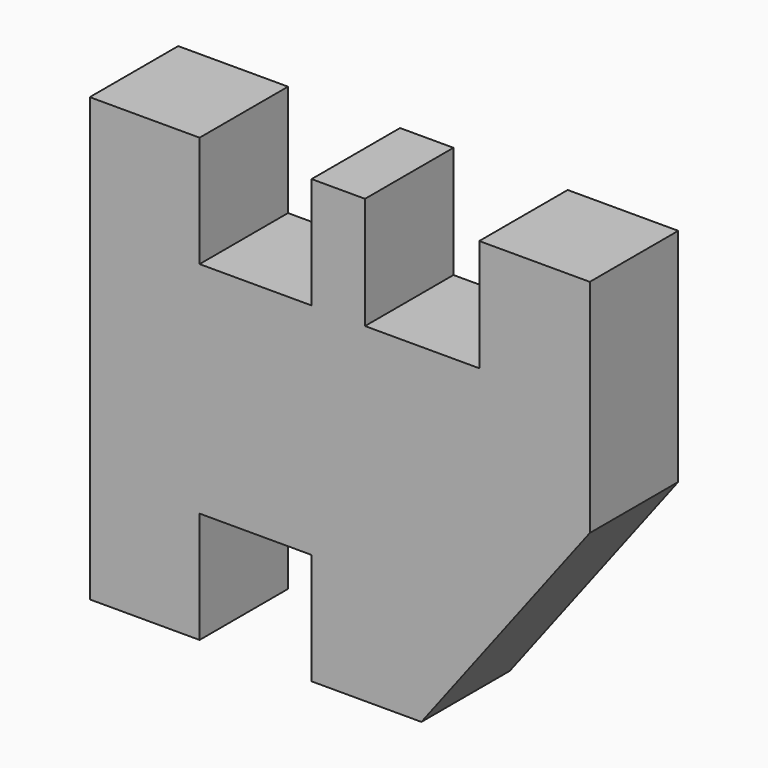
from build123d import *

# Parameters (mm, degrees)
F1_DEPTH = 3


# Not quite as in the source:
# - a feature names something its author has since deleted; it is built from what else it names


with BuildPart() as f1:
    # F0 (on Front) → F1 (new body)
    with BuildSketch(Plane.XZ):
        Polygon((1.52, 0), (4.5, 0), (9.07, 6), (9.07, 12), (6.07, 12), (6.07, 8.96), (2.97, 8.96), (2.97, 12), (1.52, 12), (1.52, 8.98), (-1.52, 8.98), (-1.52, 12), (-4.5, 12), (-4.5, 0), (-1.52, 0), (-1.52, 3.02), (1.52, 3.02), align=None)
    extrude(amount=F1_DEPTH)


solid = f1.part
